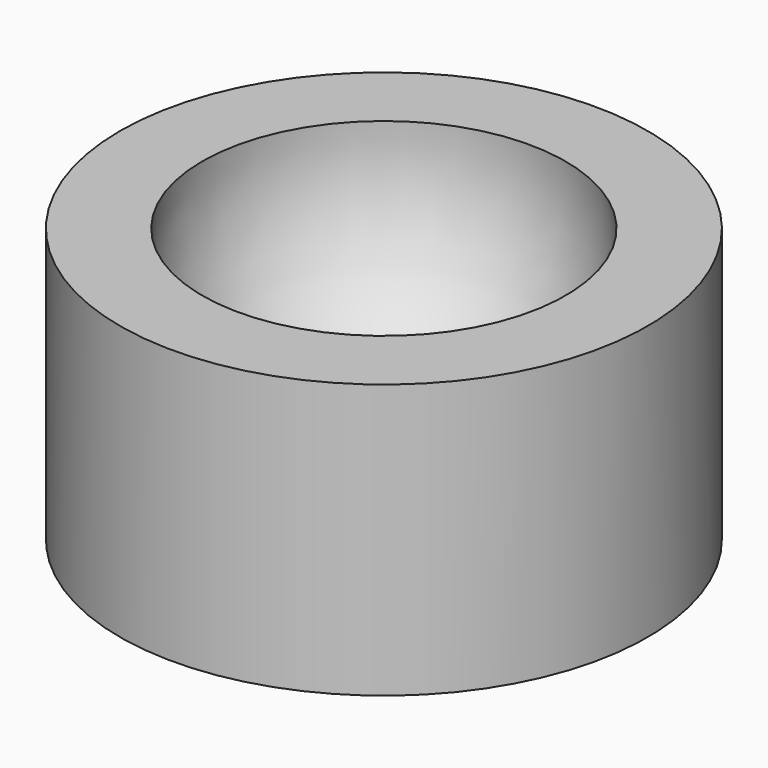
from build123d import *

# Parameters (mm, degrees)
F3_D           = 6.35
F3_CSINK_D     = 6.5
F3_CSINK_ANGLE = 90


# Not quite as in the source:
# - a feature names something its author has since deleted; it is built from what else it names


with BuildPart() as f1:
    # F0 (on Front) → F1 (revolve)
    with BuildSketch(Plane.XZ):
        with BuildLine():
            ThreePointArc((0, -14.7003533737), (-9.3251902794, -10.5563183954), (-12.4995685583, -0.8580957649))
            Line((-12.4995685583, -0.8580957649), (-18.1581123865, -0.8580957649))
            Line((-18.1581123865, -0.8580957649), (-18.1581123865, -19.7003533737))
            Line((-18.1581123865, -19.7003533737), (0, -19.7003533737))
            Line((0, -19.7003533737), (0, -14.7003533737))
        make_face()
    revolve(axis=Axis((0, 0, -17.2003533737), (0, 0, -1)))

    # F3 (through all)
    with Locations(Plane.XY):
        with Locations((0, 0)):
            CounterSinkHole(F3_D / 2, F3_CSINK_D / 2, counter_sink_angle=F3_CSINK_ANGLE)


solid = f1.part
